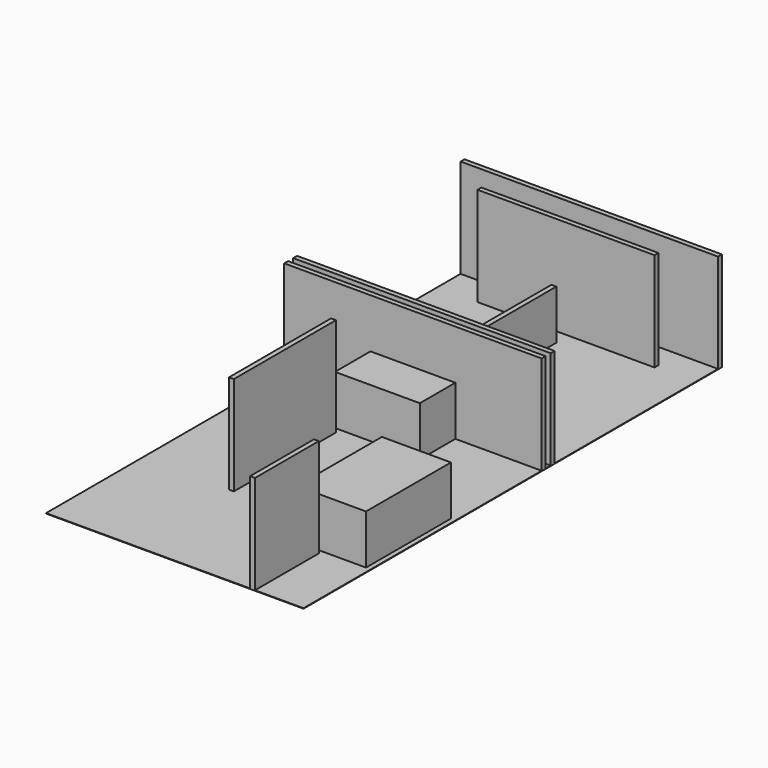
from build123d import *

# Parameters (mm, degrees)
F0_W     = 52.9098408297
F0_H     = 107.4788756669
F1_DEPTH = 0.1
F2_W     = 52.9098408297
F2_H     = 1
F3_DEPTH = 20.32
F2_W_2   = 36.3767435774
F2_W_3   = 1
F2_H_2   = 26.2354757977
F2_H_3   = 16.3882337511
F2_H_4   = 29.3569701103
F4_DEPTH = 10.16
F2_W_4   = 17.4434864894
F2_H_5   = 9.1168937506


# Not quite as in the source:
# - a feature names something its author has since deleted; it is built from what else it names
# - the program builds the solid bodies; features that only make, move or delete a surface that nothing else refers to are left out


with BuildPart() as f1:
    # F0 (on Top) → F1 (new body)
    with BuildSketch(Plane.XY):
        with Locations((-11.3378218375, -10.4160513729)):
            Rectangle(F0_W, F0_H)
    extrude(amount=F1_DEPTH)


with BuildPart() as f3:
    # F2 (on face) → F3 (new body)
    with BuildSketch(Plane.XY.offset(0.1)):
        with Locations((-11.3378218375, 42.8233864605)):
            Rectangle(F2_W, F2_H)
    extrude(amount=F3_DEPTH)


with BuildPart() as f3b:
    # F2 (on face) → F3, piece 2 (new body)
    with BuildSketch(Plane.XY.offset(0.1)):
        with Locations((-11.3378218375, 36.850056529)):
            Rectangle(F2_W_2, F2_H)
    extrude(amount=F3_DEPTH)


with BuildPart() as f3c:
    # F2 (on face) → F3, piece 3 (new body)
    with BuildSketch(Plane.XY.offset(0.1)):
        Polygon((15.1170985773, -1.9911537422), (-37.7927422523, -1.9911537422), (-37.7927422523, -2.9911537422), (-20.0595650822, -2.9911537422), (-2.6160785928, -2.9911537422), (15.1170985773, -2.9911537422), align=None)
    extrude(amount=F3_DEPTH)


with BuildPart() as f3d:
    # F2 (on face) → F3, piece 4 (new body)
    with BuildSketch(Plane.XY.offset(0.1)):
        with Locations((-19.4659615755, -26.3364540243)):
            Rectangle(F2_W_3, F2_H_2)
    extrude(amount=F3_DEPTH)


with BuildPart() as f3e:
    # F2 (on face) → F3, piece 5 (new body)
    with BuildSketch(Plane.XY.offset(0.1)):
        with Locations((4.6426873542, -55.9613723308)):
            Rectangle(F2_W_3, F2_H_3)
    extrude(amount=F3_DEPTH)


with BuildPart() as f3f:
    # F2 (on face) → F3, piece 6 (new body)
    with BuildSketch(Plane.XY.offset(0.1)):
        with Locations((-11.3378218375, -0.1677915226)):
            Rectangle(F2_W, F2_H)
    extrude(amount=F3_DEPTH)


with BuildPart() as f4:
    # F2 (on face) → F4 (new body)
    with BuildSketch(Plane.XY.offset(0.1)):
        with Locations((-11.3378218375, 18.5424766348)):
            Rectangle(F2_W_3, F2_H_4)
    extrude(amount=F4_DEPTH)


with BuildPart() as f4b:
    # F2 (on face) → F4, piece 2 (new body)
    with BuildSketch(Plane.XY.offset(0.1)):
        with Locations((-11.3378218375, -7.5496006175)):
            Rectangle(F2_W_4, F2_H_5)
    extrude(amount=F4_DEPTH)


with BuildPart() as f4c:
    # F2 (on face) → F4, piece 3 (new body)
    with BuildSketch(Plane.XY.offset(0.1)):
        Polygon((14.1368384046, -25.0625275075), (2.9698581193, -25.0625275075), (-0.0619098573, -25.0625275075), (-0.0619098573, -46.8825139105), (14.1368384046, -46.8825139105), align=None)
    extrude(amount=F4_DEPTH)


solid = Compound([f1.part, f3.part, f3b.part, f3c.part, f3d.part, f3e.part, f3f.part, f4.part, f4b.part, f4c.part])
